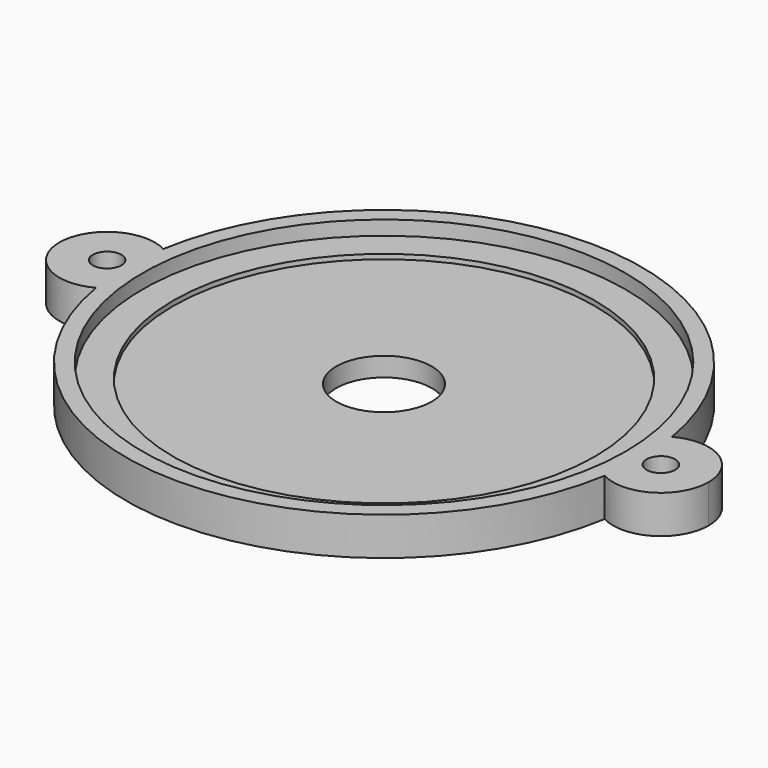
from build123d import *

# Parameters (mm, degrees)
F0_R     = 1.5
F1_DEPTH = 4
F2_DEPTH = 2
F3_R     = 27
F3_R_2   = 22.1
F4_DEPTH = 0.5
F5_R     = 25.3
F6_DEPTH = 1.5
F7_R     = 5
F8_DEPTH = 25


with BuildPart() as f1:
    # F0 (on Top) → F1 (new body)
    with BuildSketch(Plane.XY):
        with BuildLine():
            ThreePointArc((-26.6379310345, -4.4068844099), (-27, 0), (-26.6379310345, 4.4068844099))
            ThreePointArc((-26.6379310345, 4.4068844099), (-34, 0), (-26.6379310345, -4.4068844099))
        make_face()
        with Locations((-29, 0)):
            Circle(F0_R, mode=Mode.SUBTRACT)
    extrude(amount=F1_DEPTH)



with BuildPart() as f1b:
    # F0 (on Top) → F1, piece 2 (new body)
    with BuildSketch(Plane.XY):
        with BuildLine():
            ThreePointArc((26.6379310345, 4.4068844099), (26.9093305187, 2.21086658), (27, 0))
            ThreePointArc((27, 0), (26.9093305187, -2.21086658), (26.6379310345, -4.4068844099))
            ThreePointArc((26.6379310345, -4.4068844099), (31.5680396388, -4.2901249881), (34, 0))
            ThreePointArc((34, 0), (31.5680396388, 4.2901249881), (26.6379310345, 4.4068844099))
        make_face()
        with Locations((29, 0)):
            Circle(F0_R, mode=Mode.SUBTRACT)
    extrude(amount=F1_DEPTH)


with BuildPart() as f2:
    # F0 (on Top) → F2 (new body)
    with BuildSketch(Plane.XY):
        with BuildLine():
            ThreePointArc((-24, 0), (-24.7098750119, 2.5680396388), (-26.6379310345, 4.4068844099))
            ThreePointArc((-26.6379310345, 4.4068844099), (-27, 0), (-26.6379310345, -4.4068844099))
            ThreePointArc((-26.6379310345, -4.4068844099), (-24.7098750119, -2.5680396388), (-24, 0))
        make_face()
        with BuildLine():
            ThreePointArc((26.6379310345, -4.4068844099), (26.9093305187, -2.21086658), (27, 0))
            ThreePointArc((27, 0), (26.9093305187, 2.21086658), (26.6379310345, 4.4068844099))
            ThreePointArc((26.6379310345, 4.4068844099), (24, 0), (26.6379310345, -4.4068844099))
        make_face()
        with BuildLine():
            ThreePointArc((26.6379310345, -4.4068844099), (24, 0), (26.6379310345, 4.4068844099))
            ThreePointArc((26.6379310345, 4.4068844099), (0, 27), (-26.6379310345, 4.4068844099))
            ThreePointArc((-26.6379310345, 4.4068844099), (-24.7098750119, 2.5680396388), (-24, 0))
            ThreePointArc((-24, 0), (-24.7098750119, -2.5680396388), (-26.6379310345, -4.4068844099))
            ThreePointArc((-26.6379310345, -4.4068844099), (0, -27), (26.6379310345, -4.4068844099))
        make_face()
    extrude(amount=F2_DEPTH)


with BuildPart() as f1_1:
    add(f1.part)

    add(f1b.part)  # F4 merges F1b

    add(f2.part)  # F4 merges F2
    # F3 (on face) → F4 (join)
    with BuildSketch(Plane.XY.offset(2)):
        Circle(F3_R)
        Circle(F3_R_2, mode=Mode.SUBTRACT)
    extrude(amount=F4_DEPTH)

    # F5 (on face) → F6 (join)
    with BuildSketch(Plane.XY.offset(2.5)):
        with BuildLine():
            ThreePointArc((26.6379310345, -4.4068844099), (27, 0), (26.6379310345, 4.4068844099))
            ThreePointArc((26.6379310345, 4.4068844099), (0, 27), (-26.6379310345, 4.4068844099))
            ThreePointArc((-26.6379310345, 4.4068844099), (-27, 0), (-26.6379310345, -4.4068844099))
            ThreePointArc((-26.6379310345, -4.4068844099), (0, -27), (26.6379310345, -4.4068844099))
        make_face()
        Circle(F5_R, mode=Mode.SUBTRACT)
    extrude(amount=F6_DEPTH)

    # F7 (on face) → F8 (cut)
    with BuildSketch(Plane.XY.offset(2)):
        Circle(F7_R)
    extrude(amount=-F8_DEPTH, mode=Mode.SUBTRACT)


solid = f1_1.part
